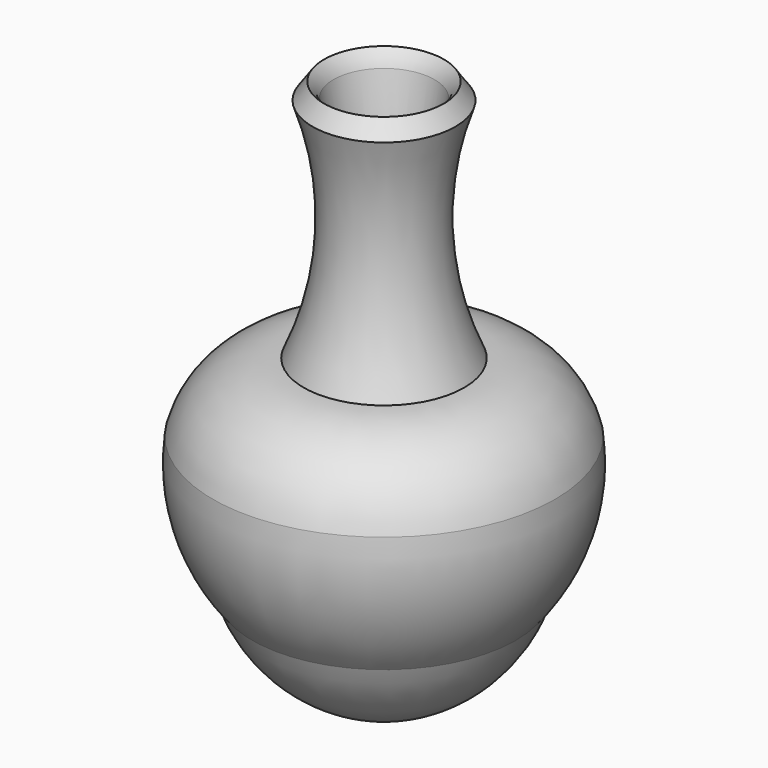
from build123d import *

# Parameters (mm, degrees)
F2_R = 5.08


# Not quite as in the source:
# - a fillet or chamfer that OpenCascade refuses, or shapes differently, is made with other operations: its cross-section is extruded or revolved along the edge and cut away or added


with BuildPart() as f1:
    # F0 (on Front) → F1 (revolve)
    with BuildSketch(Plane.XZ):
        with BuildLine():
            Line((0, -47.1050292253), (0, -50.4347011447))
            Line((0, -50.4347011447), (11.7517746985, -50.4347011447))
            ThreePointArc((11.7517746985, -50.4347011447), (20.8619938289, -43.371268105), (26.6373567283, -33.3946272731))
            ThreePointArc((26.6373567283, -33.3946272731), (33.5533359341, -20.325912086), (34.667737782, -5.5820932612))
            ThreePointArc((34.667737782, -5.5820932612), (27.9104157982, 4.6123678288), (16.2566211075, 8.3241742104))
            ThreePointArc((16.2566211075, 8.3241742104), (10.8439744561, 33.4925586358), (16.2566211075, 58.6609430611))
            Line((16.2566211075, 58.6609430611), (11.164185591, 58.6609430611))
            ThreePointArc((11.164185591, 58.6609430611), (7.8471857088, 31.7297922447), (11.164185591, 4.7986414284))
            ThreePointArc((11.164185591, 4.7986414284), (23.8420983973, 3.2667371045), (30.9463385493, -7.3448591866))
            ThreePointArc((30.9463385493, -7.3448591866), (30.5202544526, -19.8186924416), (24.6787276119, -30.8484081179))
            ThreePointArc((24.6787276119, -30.8484081179), (19.7456058465, -40.7046808706), (10.7724601403, -47.1050292253))
            Line((10.7724601403, -47.1050292253), (0, -47.1050292253))
        make_face()
    revolve(axis=Axis((0, 0, -48.769865185), (0, 0, -1)))

    # F2
    f2_edges = [f1.edges().sort_by_distance(p)[0] for p in [
        (-11.164186, 0, 58.660943),
    ]]
    fillet(f2_edges, radius=F2_R)

    # F3: chamfer of 5.08 on 1 edges, made by hand

    # F3_s1 → F3_t2 (revolve, cut)
    with BuildSketch(Plane.XZ):
        with BuildLine():
            Line((11.2721133728, 58.8272265334), (14.5927501506, 54.0993891808))
            Line((14.5927501506, 54.0993891808), (14.6883227311, 54.0649153956))
            ThreePointArc((14.6883227311, 54.0649153956), (15.3971944751, 56.3912747767), (16.3492386112, 58.6191751549))
            Line((16.3492386112, 58.6191751549), (16.2566211075, 58.7625430611))
            ThreePointArc((16.2566211075, 58.7625430611), (13.7643672402, 58.7625430611), (11.2721133728, 58.9288265334))
            Line((11.2721133728, 58.9288265334), (11.2721133728, 58.8272265334))
        make_face()
    revolve(axis=Axis((0, 0, 58.6609430611), (0, 0, -1)), mode=Mode.SUBTRACT)


solid = f1.part
